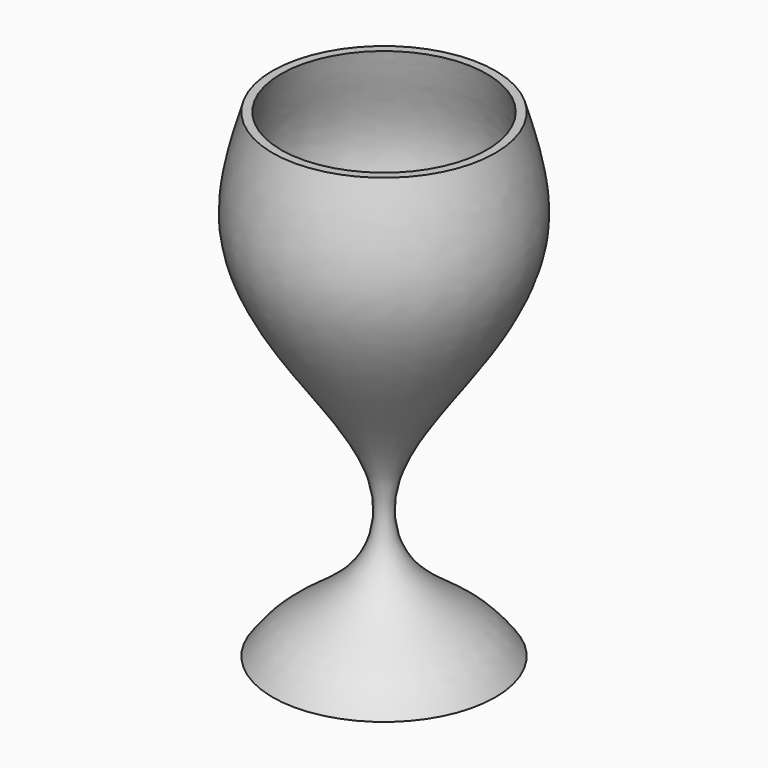
from build123d import *


with BuildPart() as f1:
    # F0 (on Front) → F1 (revolve)
    with BuildSketch(Plane.XZ):
        with BuildLine():
            Line((-26.9834566861, 10.7702212408), (-26.9834566861, 26.2599997222))
            add(Edge.make_bspline(
                [(-35.5391092598, 50.6084598601), (-35.7412288275, 49.7441475927), (-36.2258173029, 47.6719298022), (-38.1090999919, 41.8822277887), (-33.6687963717, 33.0624633891), (-29.2236970122, 28.5394879965), (-26.9834566861, 26.2599997222)],
                knots=[0, 0, 0, 0, 0.1657640951, 0.3974250046, 0.6963143689, 1, 1, 1, 1], degree=3))
            Line((-35.5391092598, 50.6084598601), (-36.2481623888, 50.6084598601))
            add(Edge.make_bspline(
                [(-36.2481623888, 10.7702212408), (-35.69477712, 11.5164713989), (-34.32820558, 13.3593181191), (-28.168588874, 16.9221381423), (-26.777434281, 24.1993426888), (-34.15823742, 33.0649179346), (-38.8219110516, 41.8988195772), (-37.0886372449, 47.7642685179), (-36.2481623888, 50.6084598601)],
                knots=[0, 0, 0, 0, 0.1083648253, 0.2676043157, 0.4218529902, 0.6278976162, 0.8195653241, 1, 1, 1, 1], degree=3))
            Line((-36.2481623888, 10.7702212408), (-26.9834566861, 10.7702212408))
        make_face()
    revolve(axis=Axis((-26.9834566861, 0, 30.6893405505), (0, 0, -1)))


solid = f1.part
